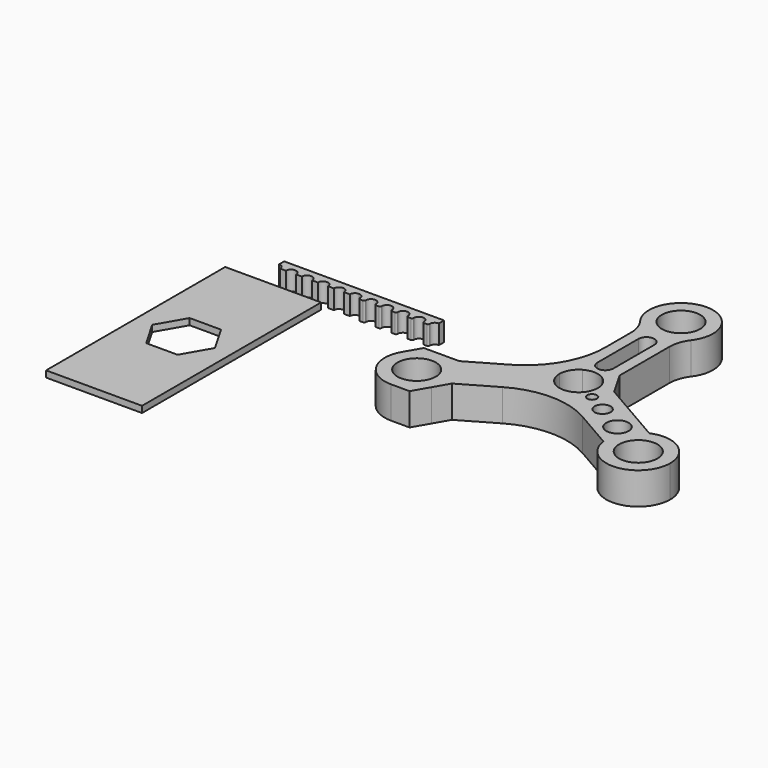
from build123d import *

# Parameters (mm, degrees)
F1_DEPTH = 6
F2_R     = 2.5
F2_R_2   = 3.5
F2_R_3   = 1.5
F3_DEPTH = 10
F4_R     = 25
F5_SIZE  = 5
F2_W     = 30
F2_H     = 70
F6_DEPTH = 2


# Not quite as in the source:
# - a feature names something its author has since deleted; it is built from what else it names


with BuildPart() as f1:
    # F0 (on Top) → F1 (new body)
    with BuildSketch(Plane.XY):
        with BuildLine():
            Line((-39.7648132003, 6.8852591163), (-37.9548132003, 6.8852591163))
            ThreePointArc((-37.9548132003, 6.8852591163), (-37.4891129824, 8.0095588984), (-36.3648132003, 8.4752591163))
            Line((-36.3648132003, 8.4752591163), (-36.3648132003, 10.4752591163))
            Line((-36.3648132003, 10.4752591163), (-61.3648132003, 10.4752591163))
            Line((-61.3648132003, 10.4752591163), (-61.3648132003, 8.4852591163))
            ThreePointArc((-61.3648132003, 8.4852591163), (-60.2334423504, 8.0166299662), (-59.7648132003, 6.8852591163))
            Line((-59.7648132003, 6.8852591163), (-57.9648132003, 6.8852591163))
            ThreePointArc((-57.9648132003, 6.8852591163), (-56.3648132003, 8.4852591163), (-54.7648132003, 6.8852591163))
            Line((-54.7648132003, 6.8852591163), (-52.9648132003, 6.8852591163))
            ThreePointArc((-52.9648132003, 6.8852591163), (-51.3648132003, 8.4852591163), (-49.7648132003, 6.8852591163))
            Line((-49.7648132003, 6.8852591163), (-47.9648132003, 6.8852591163))
            ThreePointArc((-47.9648132003, 6.8852591163), (-46.3648132003, 8.4852591163), (-44.7648132003, 6.8852591163))
            Line((-44.7648132003, 6.8852591163), (-42.9648132003, 6.8852591163))
            ThreePointArc((-42.9648132003, 6.8852591163), (-41.3648132003, 8.4852591163), (-39.7648132003, 6.8852591163))
        make_face()
        with BuildLine():
            Line((-36.3648132003, 10.4752591163), (-36.3648132003, 8.4752591163))
            ThreePointArc((-36.3648132003, 8.4752591163), (-35.2405134182, 8.0095588984), (-34.7748132003, 6.8852591163))
            Line((-34.7748132003, 6.8852591163), (-34.7748132003, 6.8152591163))
            ThreePointArc((-34.7748132003, 6.8152591163), (-34.6283665909, 6.4617057257), (-34.2748132003, 6.3152591163))
            Line((-34.2748132003, 6.3152591163), (-33.9548132003, 6.3152591163))
            Line((-33.9548132003, 6.3152591163), (-33.4548132003, 6.3152591163))
            ThreePointArc((-33.4548132003, 6.3152591163), (-33.1012598097, 6.4617057257), (-32.9548132003, 6.8152591163))
            Line((-32.9548132003, 6.8152591163), (-32.9548132003, 6.8852591163))
            ThreePointArc((-32.9548132003, 6.8852591163), (-31.3648132003, 8.4752591163), (-29.7748132003, 6.8852591163))
            Line((-29.7748132003, 6.8852591163), (-29.7748132003, 6.8152591163))
            ThreePointArc((-29.7748132003, 6.8152591163), (-29.6283665909, 6.4617057257), (-29.2748132003, 6.3152591163))
            Line((-29.2748132003, 6.3152591163), (-28.9548132003, 6.3152591163))
            Line((-28.9548132003, 6.3152591163), (-28.4548132003, 6.3152591163))
            ThreePointArc((-28.4548132003, 6.3152591163), (-28.1012598097, 6.4617057257), (-27.9548132003, 6.8152591163))
            Line((-27.9548132003, 6.8152591163), (-27.9548132003, 6.8852591163))
            ThreePointArc((-27.9548132003, 6.8852591163), (-26.3648132003, 8.4752591163), (-24.7748132003, 6.8852591163))
            Line((-24.7748132003, 6.8852591163), (-24.7748132003, 6.8152591163))
            ThreePointArc((-24.7748132003, 6.8152591163), (-24.6283665909, 6.4617057257), (-24.2748132003, 6.3152591163))
            Line((-24.2748132003, 6.3152591163), (-23.9548132003, 6.3152591163))
            Line((-23.9548132003, 6.3152591163), (-23.4548132003, 6.3152591163))
            ThreePointArc((-23.4548132003, 6.3152591163), (-23.1012598097, 6.4617057257), (-22.9548132003, 6.8152591163))
            Line((-22.9548132003, 6.8152591163), (-22.9548132003, 6.8852591163))
            ThreePointArc((-22.9548132003, 6.8852591163), (-21.3648132003, 8.4752591163), (-19.7748132003, 6.8852591163))
            Line((-19.7748132003, 6.8852591163), (-19.7748132003, 6.8152591163))
            ThreePointArc((-19.7748132003, 6.8152591163), (-19.6283665909, 6.4617057257), (-19.2748132003, 6.3152591163))
            Line((-19.2748132003, 6.3152591163), (-18.9548132003, 6.3152591163))
            Line((-18.9548132003, 6.3152591163), (-18.4548132003, 6.3152591163))
            ThreePointArc((-18.4548132003, 6.3152591163), (-18.1012598097, 6.4617057257), (-17.9548132003, 6.8152591163))
            Line((-17.9548132003, 6.8152591163), (-17.9548132003, 6.8852591163))
            ThreePointArc((-17.9548132003, 6.8852591163), (-16.3648132003, 8.4752591163), (-14.7748132003, 6.8852591163))
            Line((-14.7748132003, 6.8852591163), (-14.7748132003, 6.8152591163))
            ThreePointArc((-14.7748132003, 6.8152591163), (-14.6283665909, 6.4617057257), (-14.2748132003, 6.3152591163))
            Line((-14.2748132003, 6.3152591163), (-13.9548132003, 6.3152591163))
            Line((-13.9548132003, 6.3152591163), (-13.4548132003, 6.3152591163))
            ThreePointArc((-13.4548132003, 6.3152591163), (-13.1012598097, 6.4617057257), (-12.9548132003, 6.8152591163))
            Line((-12.9548132003, 6.8152591163), (-12.9548132003, 6.8852591163))
            ThreePointArc((-12.9548132003, 6.8852591163), (-12.4891129824, 8.0095588984), (-11.3648132003, 8.4752591163))
            Line((-11.3648132003, 8.4752591163), (-11.3648132003, 10.4752591163))
            Line((-11.3648132003, 10.4752591163), (-36.3648132003, 10.4752591163))
        make_face()
    extrude(amount=F1_DEPTH)


with BuildPart() as f3:
    # F2 (on Top) → F3 (new body)
    with BuildSketch(Plane.XY):
        with BuildLine():
            ThreePointArc((36.0828736126, 5.1961524227), (39.0828736126, 6), (42.0828736126, 5.1961524227))
            Line((42.0828736126, 5.1961524227), (45.0828736126, 3.4641016151))
            Line((45.0828736126, 3.4641016151), (45.0828736126, 28))
            ThreePointArc((45.0828736126, 28), (45.5960406321, 31.1622776602), (47.0828736126, 34))
            ThreePointArc((47.0828736126, 34), (39.0828736126, 50), (31.0828736126, 34))
            ThreePointArc((31.0828736126, 34), (32.5697065931, 31.1622776602), (33.0828736126, 28))
            Line((33.0828736126, 28), (33.0828736126, 3.4641016151))
            Line((33.0828736126, 3.4641016151), (36.0828736126, 5.1961524227))
        make_face()
        with BuildLine():
            Line((41.5828736126, 26.5050698072), (41.5828736126, 10.4311462492))
            ThreePointArc((41.5828736126, 10.4311462492), (39.0828736126, 7.9311462492), (36.5828736126, 10.4311462492))
            Line((36.5828736126, 10.4311462492), (36.5828736126, 26.5050698072))
            ThreePointArc((36.5828736126, 26.5050698072), (39.0828736126, 29.0050698072), (41.5828736126, 26.5050698072))
        make_face(mode=Mode.SUBTRACT)
        with BuildLine():
            ThreePointArc((45.0828736126, 40), (39.0828736126, 34), (33.0828736126, 40))
            ThreePointArc((33.0828736126, 40), (39.0828736126, 46), (45.0828736126, 40))
        make_face(mode=Mode.SUBTRACT)
        with BuildLine():
            ThreePointArc((36.0828736126, -5.1961524227), (33.8867211899, -3), (33.0828736126, 0))
            Line((33.0828736126, 0), (33.0828736126, 3.4641016151))
            Line((33.0828736126, 3.4641016151), (9.762365537, -10))
            Line((9.762365537, -10), (10.2153601532, -10))
            Line((10.2153601532, -10), (13.1021114244, -14.9999998707))
            Line((13.1021114244, -14.9999998707), (15.9888628451, -20))
            Line((15.9888628451, -20), (15.762365537, -20.3923048454))
            Line((15.762365537, -20.3923048454), (39.0828736126, -6.9282032303))
            Line((39.0828736126, -6.9282032303), (36.0828736126, -5.1961524227))
        make_face()
        with BuildLine():
            Line((7.4418574613, -25.1961524227), (14.3700606915, -21.1961524227))
            ThreePointArc((14.3700606915, -21.1961524227), (14.4238921312, -20.5991526088), (14.4418574613, -20))
            ThreePointArc((14.4418574613, -20), (14.1011157048, -17.4118094768), (13.1021114244, -14.9999998707))
            ThreePointArc((13.1021114244, -14.9999998707), (11.0765569379, -12.5179706727), (8.3700606915, -10.8038475773))
            Line((8.3700606915, -10.8038475773), (1.4418574613, -14.8038475773))
            ThreePointArc((1.4418574613, -14.8038475773), (7.4418574613, -14.8038475773), (10.4418574613, -20))
            ThreePointArc((10.4418574613, -20), (9.638009884, -23), (7.4418574613, -25.1961524227))
        make_face()
        with BuildLine():
            ThreePointArc((13.1021114676, -25.0000000546), (13.9286904318, -23.1622776901), (14.3700606915, -21.1961524227))
            Line((14.3700606915, -21.1961524227), (7.4418574613, -25.1961524227))
            ThreePointArc((7.4418574613, -25.1961524227), (-0.7542949614, -23), (1.4418574613, -14.8038475773))
            Line((1.4418574613, -14.8038475773), (8.3700606915, -10.8038475773))
            ThreePointArc((8.3700606915, -10.8038475773), (6.446661164, -10.2030228073), (4.4418574613, -10))
            ThreePointArc((4.4418574613, -10), (-0.5581425291, -11.3397459566), (-4.2183965654, -14.9999999807))
            ThreePointArc((-4.2183965654, -14.9999999807), (-5.5581425387, -19.9999998376), (-4.2183967279, -24.9999997379))
            ThreePointArc((-4.2183967279, -24.9999997379), (-0.5581426698, -28.6602539622), (4.4418574613, -30))
            ThreePointArc((4.4418574613, -30), (9.441857434, -28.6602540536), (13.1021114676, -25.0000000546))
        make_face()
        with BuildLine():
            Line((45.0828736126, 3.4641016151), (45.0828736126, 0))
            ThreePointArc((45.0828736126, 0), (44.2790260353, -3), (42.0828736126, -5.1961524227))
            Line((42.0828736126, -5.1961524227), (39.0828736126, -6.9282032303))
            Line((39.0828736126, -6.9282032303), (63.7956865337, -21.1961524227))
            ThreePointArc((63.7956865337, -21.1961524227), (65.0636357262, -15), (69.7956865337, -10.8038475773))
            Line((69.7956865337, -10.8038475773), (45.0828736126, 3.4641016151))
        make_face()
        with Locations((52.9936231899, -8.0313750131)):
            Circle(F2_R, mode=Mode.SUBTRACT)
        with Locations((61.6538772277, -13.0313750131)):
            Circle(F2_R_2, mode=Mode.SUBTRACT)
        with Locations((46.9314453634, -4.5313750131)):
            Circle(F2_R_3, mode=Mode.SUBTRACT)
        with BuildLine():
            ThreePointArc((83.723889764, -20), (79.2337884789, -11.6548806988), (69.7956865337, -10.8038475773))
            Line((69.7956865337, -10.8038475773), (76.723889764, -14.8038475773))
            ThreePointArc((76.723889764, -14.8038475773), (78.9200421867, -17), (79.723889764, -20))
            ThreePointArc((79.723889764, -20), (76.723889764, -25.1961524227), (70.723889764, -25.1961524227))
            Line((70.723889764, -25.1961524227), (63.7956865337, -21.1961524227))
            ThreePointArc((63.7956865337, -21.1961524227), (74.3230423728, -29.9820346699), (83.723889764, -20))
        make_face()
        with BuildLine():
            Line((76.723889764, -14.8038475773), (69.7956865337, -10.8038475773))
            ThreePointArc((69.7956865337, -10.8038475773), (65.0636357262, -15), (63.7956865337, -21.1961524227))
            Line((63.7956865337, -21.1961524227), (70.723889764, -25.1961524227))
            ThreePointArc((70.723889764, -25.1961524227), (68.5277373413, -17), (76.723889764, -14.8038475773))
        make_face()
        with BuildLine():
            Line((39.0828736126, -6.9282032303), (42.0828736126, -5.1961524227))
            ThreePointArc((42.0828736126, -5.1961524227), (39.0828736126, -6), (36.0828736126, -5.1961524227))
            Line((36.0828736126, -5.1961524227), (39.0828736126, -6.9282032303))
        make_face()
        with BuildLine():
            Line((33.0828736126, 3.4641016151), (33.0828736126, 0))
            ThreePointArc((33.0828736126, 0), (33.8867211899, 3), (36.0828736126, 5.1961524227))
            Line((36.0828736126, 5.1961524227), (33.0828736126, 3.4641016151))
        make_face()
        with BuildLine():
            ThreePointArc((42.0828736126, 5.1961524227), (44.2790260353, 3), (45.0828736126, 0))
            Line((45.0828736126, 0), (45.0828736126, 3.4641016151))
            Line((45.0828736126, 3.4641016151), (42.0828736126, 5.1961524227))
        make_face()
        with BuildLine():
            Line((10.2153601532, -10), (9.762365537, -10))
            Line((9.762365537, -10), (8.3700606915, -10.8038475773))
            ThreePointArc((8.3700606915, -10.8038475773), (11.0765569379, -12.5179706727), (13.1021114244, -14.9999998707))
            Line((13.1021114244, -14.9999998707), (10.2153601532, -10))
        make_face()
        with BuildLine():
            Line((8.3700606915, -10.8038475773), (9.762365537, -10))
            Line((9.762365537, -10), (4.4418574613, -10))
            ThreePointArc((4.4418574613, -10), (6.446661164, -10.2030228073), (8.3700606915, -10.8038475773))
        make_face()
        with BuildLine():
            ThreePointArc((-4.2183965654, -14.9999999807), (-0.5581425291, -11.3397459566), (4.4418574613, -10))
            Line((4.4418574613, -10), (-1.3316452306, -10))
            Line((-1.3316452306, -10), (-4.2183965654, -14.9999999807))
        make_face()
        with BuildLine():
            Line((14.3700606915, -21.1961524227), (15.762365537, -20.3923048454))
            Line((15.762365537, -20.3923048454), (15.9888628451, -20))
            Line((15.9888628451, -20), (13.1021114244, -14.9999998707))
            ThreePointArc((13.1021114244, -14.9999998707), (14.1011157048, -17.4118094768), (14.4418574613, -20))
            ThreePointArc((14.4418574613, -20), (14.4238921312, -20.5991526088), (14.3700606915, -21.1961524227))
        make_face()
        with BuildLine():
            Line((13.1021114676, -25.0000000546), (15.762365537, -20.3923048454))
            Line((15.762365537, -20.3923048454), (14.3700606915, -21.1961524227))
            ThreePointArc((14.3700606915, -21.1961524227), (13.9286904318, -23.1622776901), (13.1021114676, -25.0000000546))
        make_face()
        with BuildLine():
            Line((10.2153601532, -30), (13.1021114676, -25.0000000546))
            ThreePointArc((13.1021114676, -25.0000000546), (9.441857434, -28.6602540536), (4.4418574613, -30))
            Line((4.4418574613, -30), (10.2153601532, -30))
        make_face()
    extrude(amount=F3_DEPTH)

    # F4
    f4_edges = [f3.edges().sort_by_distance(p)[0] for p in [
        (33.082874, 3.464102, 5),
        (39.082874, -6.928203, 5),
    ]]
    fillet(f4_edges, radius=F4_R)

    # F5
    f5_edges = [f3.edges().sort_by_distance(p)[0] for p in [
        (45.082874, 3.464102, 5),
    ]]
    chamfer(f5_edges, length=F5_SIZE)


with BuildPart() as f6:
    # F2 (on Top) → F6 (new body)
    with BuildSketch(Plane.XY):
        with Locations((-60.5567166209, -29.8474544287)):
            Rectangle(F2_W, F2_H)
        Polygon((-70.3716711971, -29.8474544287), (-65.464193909, -21.3474544287), (-55.6492393328, -21.3474544287), (-50.7417620447, -29.8474544287), (-55.6492393328, -38.3474544287), (-65.464193909, -38.3474544287), align=None, mode=Mode.SUBTRACT)
    extrude(amount=F6_DEPTH)


solid = Compound([f1.part, f3.part, f6.part])
